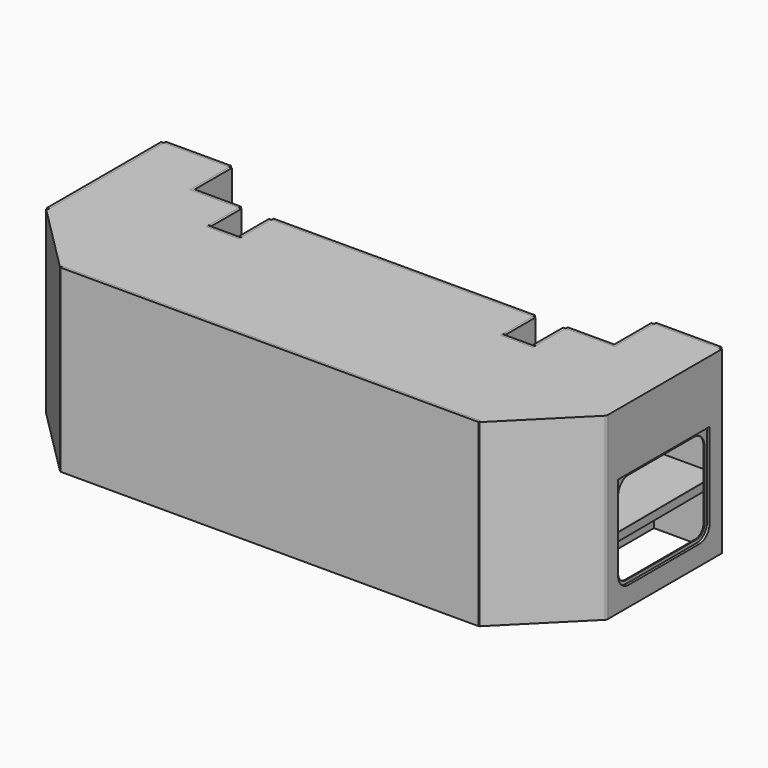
from build123d import *

# Parameters (mm, degrees)
F1_DEPTH     = 10
F3_DEPTH     = 150
F5_DEPTH     = 6
F6_W         = 437.5
F6_H         = 550
F7_DEPTH     = 8
F8_W         = 300.5203820043
F8_H         = 550
F9_DEPTH     = 8
F11_DEPTH    = 8
F12_W        = 302
F12_H        = 550
F13_DEPTH    = 8
F14_W        = 444
F14_H        = 550
F15_DEPTH    = 8
F16_W        = 200
F16_H        = 550
F17_DEPTH    = 8
F18_W        = 150
F18_H        = 550
F19_DEPTH    = 8
F20_W        = 142.0447230339
F20_H        = 550
F21_DEPTH    = 8
F22_W        = 100
F22_H        = 550
F23_DEPTH    = 8
F24_W        = 115
F24_H        = 550
F25_DEPTH    = 8
F26_W        = 115
F26_H        = 550
F27_DEPTH    = 8
F29_W        = 800
F29_H        = 550
F30_DEPTH    = 8
F31_W        = 485
F31_H        = 385
F32_DEPTH    = 8
F35_DEPTH    = 25
F37_DEPTH    = 3
F40_DEPTH    = 3
F41_W        = 439.8030777591
F41_H        = 25
F42_DEPTH    = 3
F43_W        = 1250
F43_H        = 350
F44_DEPTH    = 380
F45_T1_DEPTH = 586.5969180707


# Not quite as in the source:
# - a fillet or chamfer that OpenCascade refuses, or shapes differently, is made with other operations: its cross-section is extruded or revolved along the edge and cut away or added


with BuildPart() as f1:
    # F0 (on Top) → F1 (new body)
    with BuildSketch(Plane.XY):
        Polygon((650, 400), (650, 250), (500, 250), (500, 125), (400, 125), (400, 250), (-400, 250), (-400, 125), (-500, 125), (-500, 250), (-650, 250), (-650, 400), (-850, 400), (-850, 250), (-850, -37.5), (-637.5, -250), (637.5, -250), (850, -37.5), (850, 250), (850, 400), align=None)
    extrude(amount=-F1_DEPTH)

    # F2 (on face) → F3 (join)
    with BuildSketch(Plane(origin=(0, 0, -10), x_dir=(1, 0, 0), z_dir=(0, 0, -1))):
        Polygon((633.3578535131, 239.999973774), (-633.3578535131, 239.999973774), (-839.999973774, 33.3578535131), (-839.999973774, -389.999973774), (-660.000026226, -389.999973774), (-660.000026226, -239.999973774), (-510.000026226, -239.999973774), (-510.000026226, -114.999973774), (-389.999973774, -114.999973774), (-389.999973774, -239.999973774), (389.999973774, -239.999973774), (389.999973774, -114.999973774), (510.000026226, -114.999973774), (510.000026226, -239.999973774), (660.000026226, -239.999973774), (660.000026226, -389.999973774), (839.999973774, -389.999973774), (839.999973774, 33.3578535131), align=None)
    extrude(amount=F3_DEPTH)

    # F4 (on face) → F5 (join)
    with BuildSketch(Plane(origin=(0, 0, -160), x_dir=(1, 0, 0), z_dir=(0, 0, -1))):
        Polygon((844.999973774, -394.999973774), (844.999973774, 35.428921325), (635.428921325, 244.999973774), (-635.428921325, 244.999973774), (-844.999973774, 35.428921325), (-844.999973774, -394.999973774), (-655.000026226, -394.999973774), (-655.000026226, -244.999973774), (-505.000026226, -244.999973774), (-505.000026226, -119.999973774), (-394.999973774, -119.999973774), (-394.999973774, -244.999973774), (394.999973774, -244.999973774), (394.999973774, -119.999973774), (505.000026226, -119.999973774), (505.000026226, -244.999973774), (655.000026226, -244.999973774), (655.000026226, -394.999973774), align=None)
    extrude(amount=F5_DEPTH)

    # F8 (on face) → F9 (join)
    with BuildSketch(Plane(origin=(-443.75, -443.75, 0), x_dir=(0.7071067812, -0.7071067812, 0), z_dir=(-0.7071067812, -0.7071067812, 0))):
        with Locations((-424.2640687119, -275)):
            Rectangle(F8_W, F8_H)
    extrude(amount=F9_DEPTH)

    # F12 (on face) → F13 (join)
    with BuildSketch(Plane(origin=(443.75, -443.75, 0), x_dir=(0.7071067812, 0.7071067812, 0), z_dir=(0.7071067812, -0.7071067812, 0))):
        with Locations((423.5242597141, -275)):
            Rectangle(F12_W, F12_H)
    extrude(amount=F13_DEPTH)

    # F14 (on face) → F15 (join)
    with BuildSketch(Plane.YZ.offset(850)):
        with Locations((178, -275)):
            Rectangle(F14_W, F14_H)
    extrude(amount=F15_DEPTH)

    # F34 (on face) → F35 (cut)
    with BuildSketch(Plane.YZ.offset(858)):
        with BuildLine():
            ThreePointArc((3, -450), (14.7157287525, -478.2842712475), (43, -490))
            Line((43, -490), (313, -490))
            ThreePointArc((313, -490), (341.2842712475, -478.2842712475), (353, -450))
            Line((353, -450), (353, -190))
            Line((353, -190), (3, -190))
            Line((3, -190), (3, -450))
        make_face()
    extrude(amount=-F35_DEPTH, mode=Mode.SUBTRACT)

    # F36 (on face) → F37 (join)
    with BuildSketch(Plane(origin=(850, 0, 0), x_dir=(0, -1, 0), z_dir=(-1, 0, 0))):
        with BuildLine():
            ThreePointArc((-43, -495), (-11.1801948466, -481.8198051534), (2, -450))
            Line((2, -450), (2, -185))
            Line((2, -185), (-358, -185))
            Line((-358, -185), (-358, -450))
            ThreePointArc((-358, -450), (-344.8198051534, -481.8198051534), (-313, -495))
            Line((-313, -495), (-43, -495))
        make_face()
        with BuildLine():
            Line((-13, -240), (-13, -450))
            ThreePointArc((-13, -450), (-21.7867965644, -471.2132034356), (-43, -480))
            Line((-43, -480), (-313, -480))
            ThreePointArc((-313, -480), (-334.2132034356, -471.2132034356), (-343, -450))
            Line((-343, -450), (-343, -240))
            ThreePointArc((-343, -240), (-331.2842712475, -211.7157287525), (-303, -200))
            Line((-303, -200), (-53, -200))
            ThreePointArc((-53, -200), (-24.7157287525, -211.7157287525), (-13, -240))
        make_face(mode=Mode.SUBTRACT)
    extrude(amount=F37_DEPTH)

    # F45: fillet of radius 10 on 1 edges, made by hand

    # F45_s2 → F45_t1 (cut)
    with BuildSketch(Plane.XY.offset(-568.2984590353)):
        with BuildLine():
            ThreePointArc((858, -36.6806163859), (857.1688899271, -40.6720393784), (854.813708499, -44))
            Line((854.813708499, -44), (858, -44))
            Line((858, -44), (858, -36.6806163859))
        make_face()
    extrude(amount=F45_T1_DEPTH, mode=Mode.SUBTRACT)


with BuildPart() as f7:
    # F6 (on face) → F7 (new body)
    with BuildSketch(Plane(origin=(-850, 0, 0), x_dir=(0, -1, 0), z_dir=(-1, 0, 0))):
        with Locations((-181.25, -275)):
            Rectangle(F6_W, F6_H)
    extrude(amount=F7_DEPTH)


with BuildPart() as f11:
    # F10 (on face) → F11 (new body)
    with BuildSketch(Plane.XZ.offset(250)):
        Polygon((-637.5, 0), (-639.5, 0), (-639.5, -550), (639.5, -550), (639.5, 0), (637.5, 0), (635.5, 0), align=None)
    extrude(amount=F11_DEPTH)


with BuildPart() as f17:
    # F16 (on face) → F17 (new body)
    with BuildSketch(Plane(origin=(0, 400, 0), x_dir=(-1, 0, 0), z_dir=(0, 1, 0))):
        with Locations((750, -275)):
            Rectangle(F16_W, F16_H)
    extrude(amount=F17_DEPTH)


with BuildPart() as f19:
    # F18 (on face) → F19 (new body)
    with BuildSketch(Plane.YZ.offset(-650)):
        with Locations((325, -275)):
            Rectangle(F18_W, F18_H)
    extrude(amount=F19_DEPTH)


with BuildPart() as f21:
    # F20 (on face) → F21 (new body)
    with BuildSketch(Plane(origin=(0, 250, 0), x_dir=(-1, 0, 0), z_dir=(0, 1, 0))):
        with Locations((571.022361517, -275)):
            Rectangle(F20_W, F20_H)
    extrude(amount=F21_DEPTH)


with BuildPart() as f23:
    # F22 (on face) → F23 (new body)
    with BuildSketch(Plane(origin=(0, 125, 0), x_dir=(-1, 0, 0), z_dir=(0, 1, 0))):
        with Locations((450, -275)):
            Rectangle(F22_W, F22_H)
    extrude(amount=F23_DEPTH)


with BuildPart() as f25:
    # F24 (on face) → F25 (new body)
    with BuildSketch(Plane.YZ.offset(-500)):
        with Locations((192.5, -275)):
            Rectangle(F24_W, F24_H)
    extrude(amount=F25_DEPTH)


with BuildPart() as f27:
    # F26 (on face) → F27 (new body)
    with BuildSketch(Plane(origin=(-400, 0, 0), x_dir=(0, -1, 0), z_dir=(-1, 0, 0))):
        with Locations((-192.5, -275)):
            Rectangle(F26_W, F26_H)
    extrude(amount=F27_DEPTH)


with BuildPart() as f28_1:
    # F28: instance of F17
    add(f17.part.mirror(Plane.YZ))


with BuildPart() as f28_2:
    # F28: instance of F19
    add(f19.part.mirror(Plane.YZ))


with BuildPart() as f28_3:
    # F28: instance of F21
    add(f21.part.mirror(Plane.YZ))


with BuildPart() as f28_4:
    # F28: instance of F25
    add(f25.part.mirror(Plane.YZ))


with BuildPart() as f28_5:
    # F28: instance of F23
    add(f23.part.mirror(Plane.YZ))


with BuildPart() as f28_6:
    # F28: instance of F27
    add(f27.part.mirror(Plane.YZ))


with BuildPart() as f30:
    # F29 (on face) → F30 (new body)
    with BuildSketch(Plane(origin=(0, 250, 0), x_dir=(-1, 0, 0), z_dir=(0, 1, 0))):
        with Locations((0, -275)):
            Rectangle(F29_W, F29_H)
    extrude(amount=F30_DEPTH)


with BuildPart() as f32:
    # F31 (on face) → F32 (new body)
    with BuildSketch(Plane(origin=(-650, 0, 0), x_dir=(0, -1, 0), z_dir=(-1, 0, 0))):
        with Locations((-7.5, -357.5)):
            Rectangle(F31_W, F31_H)
    extrude(amount=-F32_DEPTH)


with BuildPart() as f33_1:
    # F33: instance of F32
    add(f32.part.mirror(Plane.YZ))


with BuildPart() as f40:
    # F39 (on offset) → F40 (new body)
    with BuildSketch(Plane(origin=(0, 0, -341), x_dir=(1, 0, 0), z_dir=(0, 0, -1))):
        Polygon((654.4221624106, 231.1809549509), (650.6431698799, -399.4338214397), (844.8856899004, -399.4338214397), (847.5211858749, 40.3613597155), align=None)
    extrude(amount=F40_DEPTH)


with BuildPart() as f42:
    # F41 (on face) → F42 (new body)
    with BuildSketch(Plane(origin=(847.2488929893, 5.0771839769, 0), x_dir=(-0.0059924455, 0.9999820451, 0), z_dir=(0.9999820451, 0.0059924455, 0))):
        with Locations((174.4621793297, -353.5)):
            Rectangle(F41_W, F41_H)
    extrude(amount=-F42_DEPTH)


with BuildPart() as f44:
    # F43 (on face) → F44 (new body)
    with BuildSketch(Plane(origin=(0, 0, -166), x_dir=(1, 0, 0), z_dir=(0, 0, -1))):
        with Locations((0, 62.499973774)):
            Rectangle(F43_W, F43_H)
    extrude(amount=F44_DEPTH)


solid = Compound([f1.part, f7.part, f11.part, f17.part, f19.part, f21.part, f23.part, f25.part, f27.part, f28_1.part, f28_2.part, f28_3.part, f28_4.part, f28_5.part, f28_6.part, f30.part, f32.part, f33_1.part, f40.part, f42.part, f44.part])
